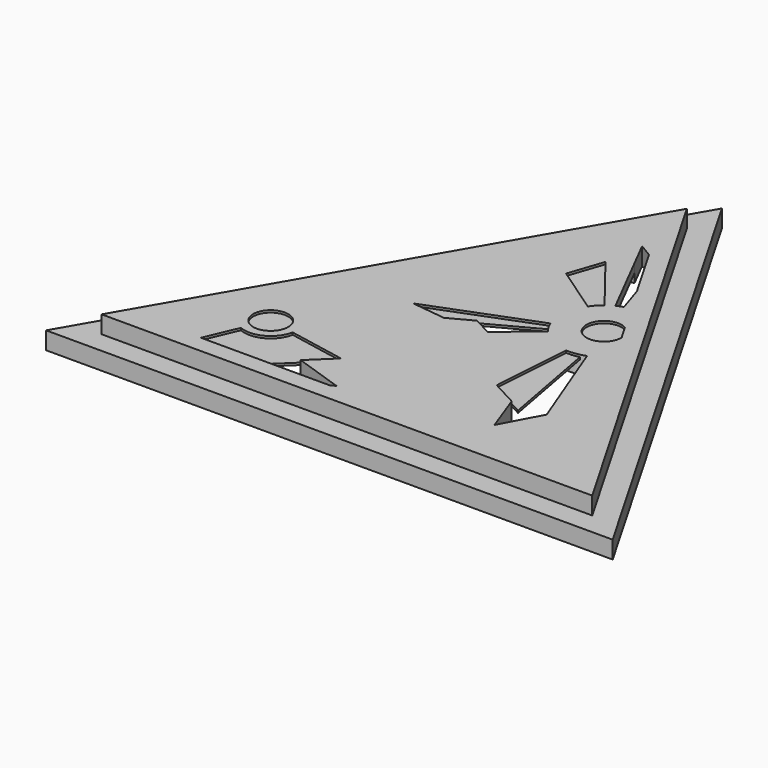
from build123d import *

# Parameters (mm, degrees)
F1_DEPTH  = 4
F2_DEPTH  = 2
F3_START  = 2
F3_DEPTH  = 2
F4_SIZE   = 1.99999
F6_START  = 3.75
F5_R      = 2
F6_DEPTH  = 0.25
F7_DEPTH  = 3.5
F8_DEPTH  = 3.5
F9_DEPTH  = 3
F10_DEPTH = 3.25
F11_DEPTH = 3


# Not quite as in the source:
# - a fillet or chamfer is up to 0.001 mm smaller than in the source, because OpenCascade refuses the exact size


with BuildPart() as f1:
    # F0 (on Top) → F1 (new body)
    with BuildSketch(Plane.XY):
        Polygon((32.7846783229, 14.824549064), (4.8026783229, 63.2907947614), (-23.1793216771, 14.824549064), align=None)
        Polygon((-19.715220062, 16.824549064), (4.8026783229, 59.2907947614), (29.3205767077, 16.824549064), align=None, mode=Mode.SUBTRACT)
    extrude(amount=F1_DEPTH)

    # F0 (on Top) → F2 (join)
    with BuildSketch(Plane.XY):
        Polygon((37.1148053418, 12.324549064), (4.8026783229, 68.2907947614), (-27.509448696, 12.324549064), align=None)
        Polygon((-23.1793216771, 14.824549064), (4.8026783229, 63.2907947614), (32.7846783229, 14.824549064), align=None, mode=Mode.SUBTRACT)
    extrude(amount=F2_DEPTH)

    # F0 (on Top) → F3 (join)
    with BuildSketch(Plane.XY.offset(F3_START)):
        Polygon((29.3205767077, 16.824549064), (4.8026783229, 59.2907947614), (-19.715220062, 16.824549064), align=None)
    extrude(amount=F3_DEPTH)

    # F4 (size 2 in the source; OpenCascade refuses exactly that, so slightly less here)
    f4_edges = [f1.edges().sort_by_distance(p)[0] for p in [
        (4.802678, 16.824549, 0),
        (-7.456271, 38.057672, 0),
        (17.061628, 38.057672, 0),
    ]]
    chamfer(f4_edges, length=F4_SIZE)

    # F5 (on face) → F6 (cut)
    with BuildSketch(Plane.XY.offset(F6_START)):
        with BuildLine():
            Line((15.8012454512, 40.2407176847), (14.8071694273, 41.9625078646))
            ThreePointArc((14.8071694273, 41.9625078646), (12.0675004242, 39.2368445398), (15.801257126, 40.2338840067))
            ThreePointArc((15.801257126, 40.2338840067), (15.8012542073, 40.2373008507), (15.8012454512, 40.2407176847))
        make_face()
        with BuildLine():
            Line((17.0693753854, 23.8813530259), (14.9441122519, 35.3662478082))
            ThreePointArc((14.9441122519, 35.3662478082), (14.2087911946, 35.2505200844), (13.4644377158, 35.2452416378))
            Line((13.4644377158, 35.2452416378), (12.8494622186, 26.1368211359))
            Line((12.8494622186, 26.1368211359), (15.8132929355, 24.552706629))
            Line((15.8132929355, 24.552706629), (17.0693753854, 23.8813530259))
        make_face()
        with BuildLine():
            ThreePointArc((9.6781818277, 43.0623553402), (10.154568974, 43.6546537332), (10.7152328484, 44.1678964823))
            Line((10.7152328484, 44.1678964823), (5.5434275419, 50.7608279586))
            Line((5.5434275419, 50.7608279586), (5.1609951292, 49.6271412781))
            Line((5.1609951292, 49.6271412781), (4.2115291581, 46.8125343323))
            Line((4.2115291581, 46.8125343323), (9.6781818277, 43.0623553402))
        make_face()
        with BuildLine():
            Line((-13.4587365793, 16.824549064), (-6.1025659626, 16.824549064))
            Line((-6.1025659626, 16.824549064), (-3.819498702, 19.0105444595))
            Line((-3.819498702, 19.0105444595), (-1.2189327972, 21.5005390346))
            Line((-1.2189327972, 21.5005390346), (-7.725601985, 22.742720621))
            ThreePointArc((-7.725601985, 22.742720621), (-9.2656609828, 20.6555454959), (-11.8573356204, 20.5492238495))
            Line((-11.8573356204, 20.5492238495), (-13.4587365793, 16.824549064))
        make_face()
        with BuildLine():
            Line((3.6860700174, 34.755180139), (9.4204377363, 37.8238173116))
            ThreePointArc((9.4204377363, 37.8238173116), (9.2694965624, 38.1212680469), (9.1387235678, 38.4281207834))
            Line((9.1387235678, 38.4281207834), (0.9941436583, 35.2838113904))
            Line((0.9941436583, 35.2838113904), (-2.8154677711, 33.8130667806))
            Line((-2.8154677711, 33.8130667806), (1.0452440474, 33.3419926465))
            Line((1.0452440474, 33.3419926465), (3.6860700174, 34.755180139))
        make_face()
        with Locations((-10.6723830104, 23.3052875847)):
            Circle(F5_R)
    extrude(amount=F6_DEPTH, mode=Mode.SUBTRACT)

    # F5 (on face) → F7 (cut)
    with BuildSketch(Plane.XY):
        with BuildLine():
            Line((15.8012454512, 40.2407176847), (14.8071694273, 41.9625078646))
            ThreePointArc((14.8071694273, 41.9625078646), (12.0675004242, 39.2368445398), (15.801257126, 40.2338840067))
            ThreePointArc((15.801257126, 40.2338840067), (15.8012542073, 40.2373008507), (15.8012454512, 40.2407176847))
        make_face()
        with Locations((-10.6723830104, 23.3052875847)):
            Circle(F5_R)
    extrude(amount=F7_DEPTH, mode=Mode.SUBTRACT)

    # F5 (on face) → F8 (cut)
    with BuildSketch(Plane.XY):
        with BuildLine():
            Line((3.6860700174, 34.755180139), (9.4204377363, 37.8238173116))
            ThreePointArc((9.4204377363, 37.8238173116), (9.2694965624, 38.1212680469), (9.1387235678, 38.4281207834))
            Line((9.1387235678, 38.4281207834), (0.9941436583, 35.2838113904))
            Line((0.9941436583, 35.2838113904), (-2.8154677711, 33.8130667806))
            Line((-2.8154677711, 33.8130667806), (1.0452440474, 33.3419926465))
            Line((1.0452440474, 33.3419926465), (3.6860700174, 34.755180139))
        make_face()
        with BuildLine():
            Line((17.0693753854, 23.8813530259), (14.9441122519, 35.3662478082))
            ThreePointArc((14.9441122519, 35.3662478082), (14.2087911946, 35.2505200844), (13.4644377158, 35.2452416378))
            Line((13.4644377158, 35.2452416378), (12.8494622186, 26.1368211359))
            Line((12.8494622186, 26.1368211359), (15.8132929355, 24.552706629))
            Line((15.8132929355, 24.552706629), (17.0693753854, 23.8813530259))
        make_face()
        with BuildLine():
            Line((-13.4587365793, 16.824549064), (-6.1025659626, 16.824549064))
            Line((-6.1025659626, 16.824549064), (-3.819498702, 19.0105444595))
            Line((-3.819498702, 19.0105444595), (-1.2189327972, 21.5005390346))
            Line((-1.2189327972, 21.5005390346), (-7.725601985, 22.742720621))
            ThreePointArc((-7.725601985, 22.742720621), (-9.2656609828, 20.6555454959), (-11.8573356204, 20.5492238495))
            Line((-11.8573356204, 20.5492238495), (-13.4587365793, 16.824549064))
        make_face()
        with BuildLine():
            ThreePointArc((9.6781818277, 43.0623553402), (10.154568974, 43.6546537332), (10.7152328484, 44.1678964823))
            Line((10.7152328484, 44.1678964823), (5.5434275419, 50.7608279586))
            Line((5.5434275419, 50.7608279586), (5.1609951292, 49.6271412781))
            Line((5.1609951292, 49.6271412781), (4.2115291581, 46.8125343323))
            Line((4.2115291581, 46.8125343323), (9.6781818277, 43.0623553402))
        make_face()
    extrude(amount=F8_DEPTH, mode=Mode.SUBTRACT)

    # F5 (on face) → F9 (cut)
    with BuildSketch(Plane.XY):
        with BuildLine():
            Line((19.8564007878, 24.4885329157), (15.5959561349, 35.5670804467))
            ThreePointArc((15.5959561349, 35.5670804467), (15.2734627879, 35.4555359146), (14.9441122519, 35.3662478082))
            Line((14.9441122519, 35.3662478082), (17.0693753854, 23.8813530259))
            Line((17.0693753854, 23.8813530259), (15.8132929355, 24.552706629))
            Line((15.8132929355, 24.552706629), (17.4690298736, 20.0315453112))
            Line((17.4690298736, 20.0315453112), (19.8564007878, 24.4885329157))
        make_face()
        Polygon((-6.1025659626, 16.824549064), (1.2875116271, 16.824549064), (1.7734020948, 17.1169545501), (-3.819498702, 19.0105444595), align=None)
        with BuildLine():
            Line((5.785849411, 33.66388008), (9.9342960343, 37.064244924))
            ThreePointArc((9.9342960343, 37.064244924), (9.6599157648, 37.4322252607), (9.4204377363, 37.8238173116))
            Line((9.4204377363, 37.8238173116), (3.6860700174, 34.755180139))
            Line((3.6860700174, 34.755180139), (5.785849411, 33.66388008))
        make_face()
        with BuildLine():
            ThreePointArc((11.5326481984, 44.6896009562), (11.8941525727, 44.8558913869), (12.2677356256, 44.9929082563))
            Line((12.2677356256, 44.9929082563), (11.2701070238, 48.0888796571))
            Line((11.2701070238, 48.0888796571), (7.7075759005, 54.2593645662))
            Line((7.7075759005, 54.2593645662), (6.1958078295, 55.1715530455))
            Line((6.1958078295, 55.1715530455), (7.7216781624, 52.1746300315))
            Line((7.7216781624, 52.1746300315), (11.5326481984, 44.6896009562))
        make_face()
        with BuildLine():
            ThreePointArc((-12.7082549566, 21.1018299793), (-12.079105038, 25.9550296735), (-7.7066088949, 23.7571547066))
            Line((-7.7066088949, 23.7571547066), (-6.6805827438, 23.5612770993))
            ThreePointArc((-6.6805827438, 23.5612770993), (-12.5480123805, 26.8382770364), (-13.1208381636, 20.1422088056))
            Line((-13.1208381636, 20.1422088056), (-12.7082549566, 21.1018299793))
        make_face()
    extrude(amount=F9_DEPTH, mode=Mode.SUBTRACT)

    # F10 (cut): faces of the model
    f10_faces = [f1.faces().sort_by_distance(p)[0] for p in [
        (9.5592668565, 49.7626778986, 3),
        (6.8730240158, 35.6258562625, 3),
        (-2.519612135, 17.5665266523, 3),
        (17.3422888297, 27.0693911728, 3),
    ]]
    extrude(f10_faces, amount=-F10_DEPTH, mode=Mode.SUBTRACT)

    # F5 (on face) → F11 (cut)
    with BuildSketch(Plane.XY):
        with BuildLine():
            ThreePointArc((9.1387235678, 38.4281207834), (8.9697402045, 38.9468547775), (8.8582790135, 39.4809116441))
            Line((8.8582790135, 39.4809116441), (1.4540485572, 38.196541369))
            Line((1.4540485572, 38.196541369), (0.9941436583, 35.2838113904))
            Line((0.9941436583, 35.2838113904), (9.1387235678, 38.4281207834))
        make_face()
        with BuildLine():
            ThreePointArc((10.7152328484, 44.1678964823), (11.1112630591, 44.4486119837), (11.5326481984, 44.6896009562))
            Line((11.5326481984, 44.6896009562), (7.7216781624, 52.1746300315))
            Line((7.7216781624, 52.1746300315), (3.6355266348, 51.2855537236))
            Line((3.6355266348, 51.2855537236), (5.1609951292, 49.6271412781))
            Line((5.1609951292, 49.6271412781), (5.5434275419, 50.7608279586))
            Line((5.5434275419, 50.7608279586), (10.7152328484, 44.1678964823))
        make_face()
    extrude(amount=F11_DEPTH, mode=Mode.SUBTRACT)


solid = f1.part
